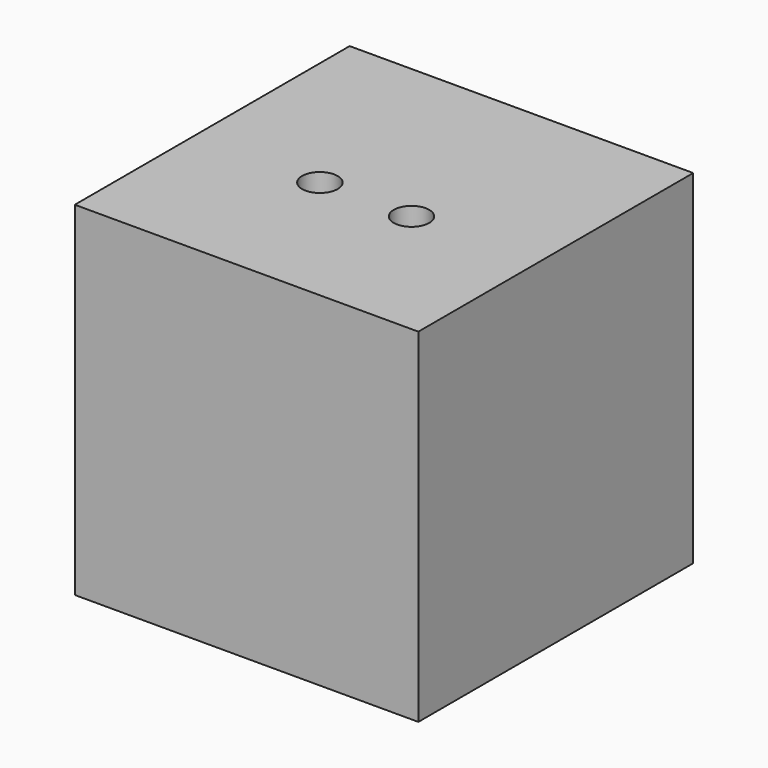
from build123d import *

# Parameters (mm, degrees)
F0_W     = 30
F0_H     = 30
F1_DEPTH = 30
F2_R     = 1.55
F3_DEPTH = 6


# Not quite as in the source:
# - a feature names something its author has since deleted; it is built from what else it names


with BuildPart() as f1:
    # F0 (on Top) → F1 (new body)
    with BuildSketch(Plane.XY):
        Rectangle(F0_W, F0_H)
    extrude(amount=F1_DEPTH)

    # F2 (on face) → F3 (cut)
    with BuildSketch(Plane.XY.offset(30)):
        with Locations((-4, -2)):
            Circle(F2_R)
        with Locations((4, -2)):
            Circle(F2_R)
    extrude(amount=-F3_DEPTH, mode=Mode.SUBTRACT)


solid = f1.part
